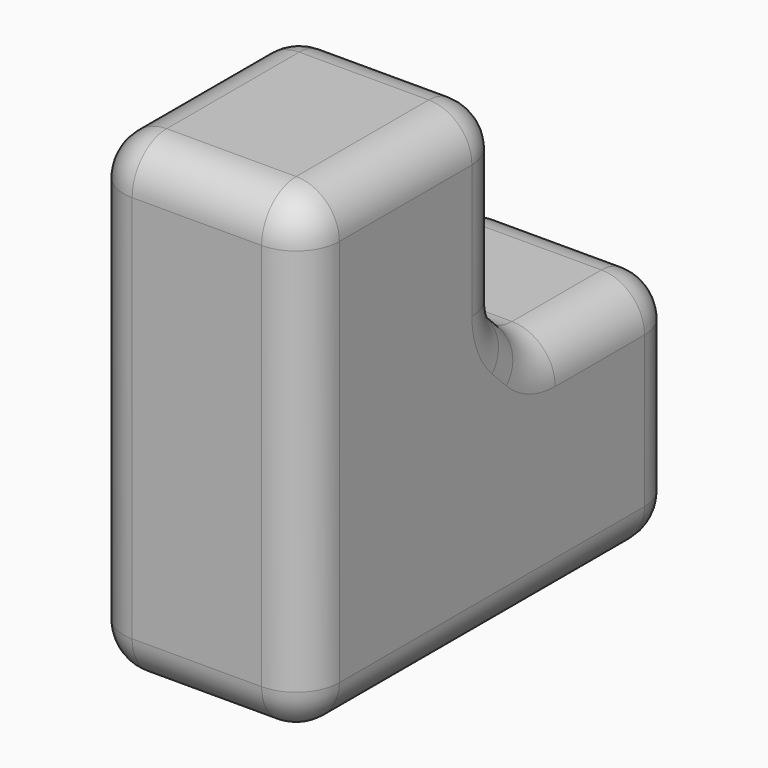
from build123d import *

# Parameters (mm, degrees)
F0_W     = 25.4
F0_H     = 27.94
F1_DEPTH = 25.4
F2_SIZE  = 5.08
F3_F1_R  = 5.08
F3_F2_R  = 5.08


with BuildPart() as f1:
    # F0 (on Right) → F1 (new body)
    with BuildSketch(Plane.YZ):
        Polygon((-14.8341231188, -27.94), (14.8341231188, -27.94), (14.8341231188, 0), (14.8341231188, 27.94), (-14.8341231188, 27.94), align=None)
        with Locations((27.5341231188, -13.97)):
            Rectangle(F0_W, F0_H)
    extrude(amount=F1_DEPTH)

    # F2
    f2_edges = [f1.edges().sort_by_distance(p)[0] for p in [
        (12.7, 14.834123, 0),
    ]]
    chamfer(f2_edges, length=F2_SIZE)

    # F3: fillet of radius 5.08 on 20 edges, made by hand

    # F3_f1
    f3_f1_edges = [f1.edges().sort_by_distance(p)[0] for p in [
        (12.7, 14.8341231188, 5.08),
        (12.7, 19.9141231188, 0),
    ]]
    fillet(f3_f1_edges, radius=F3_F1_R)

    # F3_f2
    f3_f2_edges = [f1.edges().sort_by_distance(p)[0] for p in [
        (12.7, 14.8341231188, 27.94),
        (25.4, 14.8341231188, 17.5621024484),
        (25.4, 0, 27.94),
        (12.7, -14.8341231188, 27.94),
        (0, 0, 27.94),
        (25.4, -14.8341231188, 0),
        (25.4, 12.7, -27.94),
        (25.4, 31.1262255672, 0),
        (25.4, 40.2341231188, -13.97),
        (12.7, 40.2341231188, 0),
        (0, 31.1262255672, 0),
        (0, 40.2341231188, -13.97),
        (12.7, 40.2341231188, -27.94),
        (0, 17.3741231188, 2.54),
        (25.4, 17.3741231188, 2.54),
        (0, 12.7, -27.94),
        (0, -14.8341231188, 0),
        (12.7, -14.8341231188, -27.94),
        (25.4, 20.0742961792, 0.3866919748),
        (25.4, 15.2208150936, 5.2401730604),
        (0, 20.0742961792, 0.3866919748),
        (0, 15.2208150936, 5.2401730604),
    ]]
    fillet(f3_f2_edges, radius=F3_F2_R)


solid = f1.part
